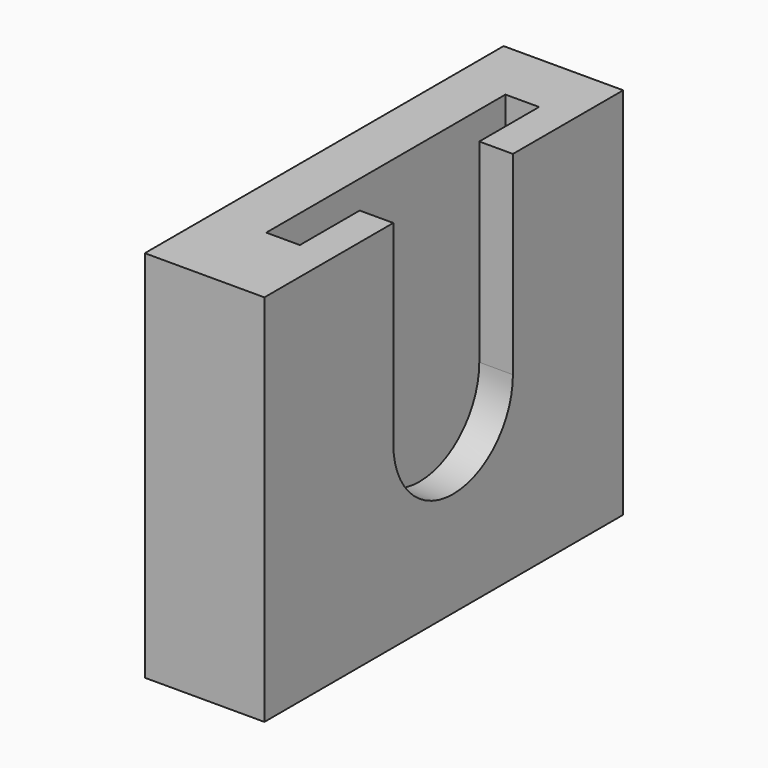
from build123d import *

# Parameters (mm, degrees)
F0_W     = 8
F0_H     = 30
F1_DEPTH = 25
F5_DEPTH = 2.25
F7_DEPTH = 2.251


# Not quite as in the source:
# - a feature of the source that left no trace in its solid (it failed there, or was rolled back) is left out


with BuildPart() as f1:
    # F0 (on Top) → F1 (new body)
    with BuildSketch(Plane.XY):
        with Locations((4.3632484525, -0.778583717)):
            Rectangle(F0_W, F0_H)
    extrude(amount=F1_DEPTH)

    # F4 (on offset) → F5 (cut, through all)
    with BuildSketch(Plane.YZ.offset(3.8632484525)):
        with BuildLine():
            Line((-10, 26.291980999), (-10, 12))
            ThreePointArc((-10, 12), (0, 2), (10, 12))
            Line((10, 12), (10, 26.291980999))
            Line((10, 26.291980999), (-10, 26.291980999))
        make_face()
    extrude(amount=F5_DEPTH, mode=Mode.SUBTRACT)

    # F6 (on offset) → F7 (cut, through all)
    with BuildSketch(Plane.YZ.offset(6.1132484525)):
        with BuildLine():
            Line((-5, 26.8745111924), (-5, 12))
            ThreePointArc((-5, 12), (0, 7), (5, 12))
            Line((5, 12), (5, 26.8745111924))
            Line((5, 26.8745111924), (-5, 26.8745111924))
        make_face()
    extrude(amount=F7_DEPTH, mode=Mode.SUBTRACT)


solid = f1.part
